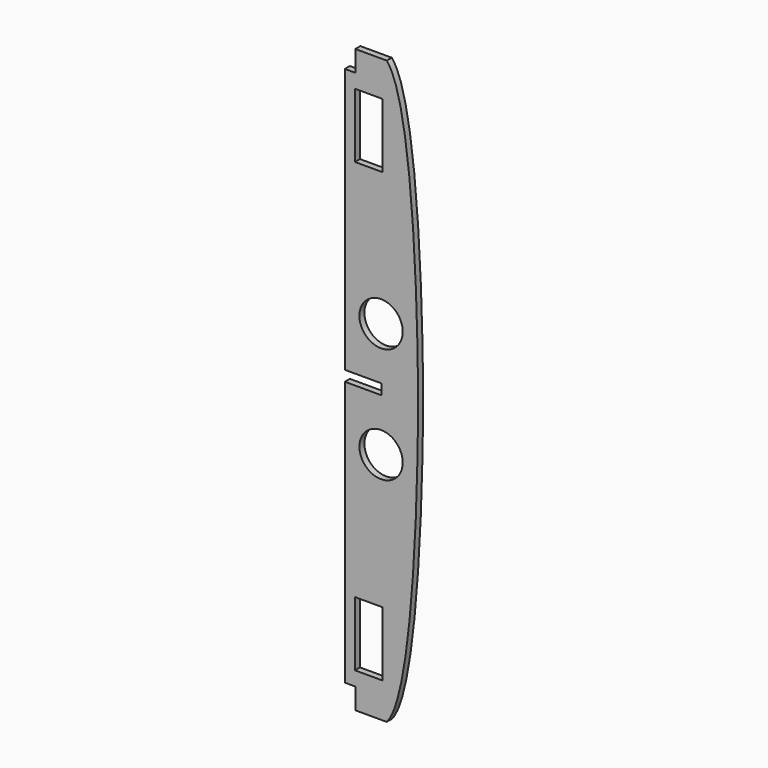
from build123d import *

# Parameters (mm, degrees)
F0_W     = 26.264000684
F0_H     = 61.5584850311
F0_R     = 20.6845185899
F1_DEPTH = 6


# Not quite as in the source:
# - a feature names something its author has since deleted; it is built from what else it names


with BuildPart() as f1:
    # F0 (on Front) → F1 (new body)
    with BuildSketch(Plane.XZ):
        with BuildLine():
            Line((-85.3373999149, -282.300586921), (-55.3373999149, -282.300586921))
            add(Edge.make_bspline(
                [(-55.3373999149, -282.300586921), (-25.3373999149, -248.5114336432), (-25.3373999149, -8.6011738421), (-25.3373999149, -4.300586921)],
                knots=[0, 0, 0, 0, 279.6140196771, 279.6140196771, 279.6140196771, 279.6140196771], degree=3))
            Line((-25.3373999149, -4.300586921), (-52.1773999149, -4.300586921))
            Line((-52.1773999149, -4.300586921), (-60.3373999149, -4.300586921))
            Line((-60.3373999149, -4.300586921), (-60.3373999149, -9.300586921))
            Line((-60.3373999149, -9.300586921), (-95.3373999149, -9.300586921))
            Line((-95.3373999149, -9.300586921), (-95.3373999149, -262.300586921))
            Line((-95.3373999149, -262.300586921), (-85.3373999149, -262.300586921))
            Line((-85.3373999149, -262.300586921), (-85.3373999149, -282.300586921))
        make_face()
        with Locations((-72.504458949, -217.9853469969)):
            Rectangle(F0_W, F0_H, mode=Mode.SUBTRACT)
        with Locations((-60.7578158379, -59.3237542452)):
            Circle(F0_R, mode=Mode.SUBTRACT)
        Polygon((-52.1773999149, -4.300586921), (-25.3373999149, -4.300586921), (-25.3373999149, 273.699413079), (-55.3373999149, 273.699413079), (-85.3373999149, 273.699413079), (-85.3373999149, 253.699413079), (-95.3373999149, 253.699413079), (-95.3373999149, 0.699413079), (-60.3373999149, 0.699413079), (-60.3373999149, -4.300586921), align=None)
        with Locations((-60.7578158379, 50.7225804031)):
            Circle(F0_R, mode=Mode.SUBTRACT)
        with Locations((-72.504458949, 209.3841731548)):
            Rectangle(F0_W, F0_H, mode=Mode.SUBTRACT)
        with BuildLine():
            add(Edge.make_bspline(
                [(-55.3373999149, 273.699413079), (-25.3373999149, 239.9102598011), (-25.3373999149, 0), (-25.3373999149, -4.300586921)],
                knots=[0, 0, 0, 0, 279.6140196771, 279.6140196771, 279.6140196771, 279.6140196771], degree=3))
            Line((-55.3373999149, 273.699413079), (-25.3373999149, 273.699413079))
            Line((-25.3373999149, 273.699413079), (-25.3373999149, -4.300586921))
        make_face(mode=Mode.SUBTRACT)
    extrude(amount=F1_DEPTH)


solid = f1.part
